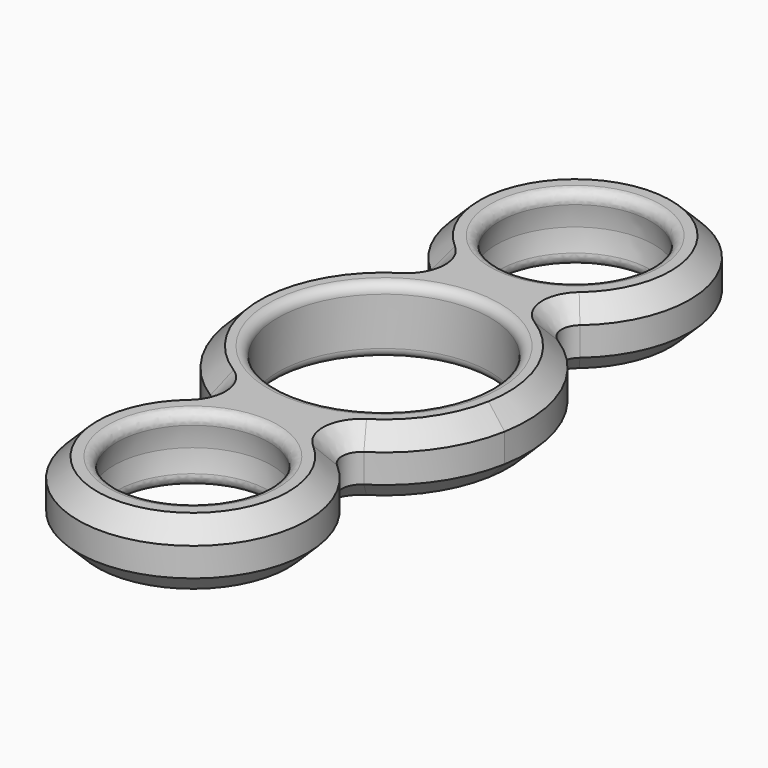
from build123d import *

# Parameters (mm, degrees)
F0_R     = 8.25
F0_R_2   = 11.1
F1_DEPTH = 7
F2_R     = 2
F3_SIZE  = 2
F9_R     = 1


# Not quite as in the source:
# - a pattern or mirror of a feature is missing from the dataset's text; its kind, count and spacing are read off the source's solid
# - a feature names something its author has since deleted; it is built from what else it names


with BuildPart() as f1:
    # F0 (on Top) → F1 (new body)
    with BuildSketch(Plane.XY):
        with BuildLine():
            ThreePointArc((14.7593654246, -2.6760291972), (12.9903810568, 7.5), (5.0621734463, 14.12))
            ThreePointArc((5.0621734463, 14.12), (0, 37), (-5.0621734463, 14.12))
            ThreePointArc((-5.0621734463, 14.12), (-15, 0), (-5.0621734463, -14.12))
            ThreePointArc((-5.0621734463, -14.12), (0, -37), (5.0621734463, -14.12))
            ThreePointArc((5.0621734463, -14.12), (11.4439708028, -9.6971919783), (14.7593654246, -2.6760291972))
        make_face()
        with Locations((0, -25)):
            Circle(F0_R, mode=Mode.SUBTRACT)
        Circle(F0_R_2, mode=Mode.SUBTRACT)
        with Locations((0, 25)):
            Circle(F0_R, mode=Mode.SUBTRACT)
    extrude(amount=F1_DEPTH)

    # F2
    f2_edges = [f1.edges().sort_by_distance(p)[0] for p in [
        (5.062173, -14.12, 3.5),
        (5.062173, 14.12, 3.5),
        (-5.062173, 14.12, 3.5),
        (-5.062173, -14.12, 3.5),
    ]]
    fillet(f2_edges, radius=F2_R)

    # F3
    f3_edges = [f1.edges().sort_by_distance(p)[0] for p in [
        (0, -37, 7),
        (0, -37, 0),
        (15, 0, 7),
        (15, 0, 0),
        (7.104012, 14.217419, 7),
        (7.104012, -14.217419, 7),
        (0, 37, 7),
        (-7.104012, 14.217419, 7),
        (-7.104012, -14.217419, 7),
        (-15, 0, 7),
        (7.104012, 14.217419, 0),
        (7.104012, -14.217419, 0),
        (0, 37, 0),
        (-7.104012, -14.217419, 0),
        (-7.104012, 14.217419, 0),
        (-15, 0, 0),
    ]]
    chamfer(f3_edges, length=F3_SIZE)

    # F7 (on 3pt) → F8 (revolve)
    with BuildSketch(Plane.YZ):
        with BuildLine():
            Line((-32.4707763987, 7), (-33.25, 7))
            Line((-33.25, 7), (-33.25, 3.5))
            ThreePointArc((-33.25, 3.5), (-33.0528381733, 5.2928461605), (-32.4707763987, 7))
        make_face()
        with BuildLine():
            ThreePointArc((-32.4707763987, 0), (-33.0528381733, 1.7071538395), (-33.25, 3.5))
            Line((-33.25, 3.5), (-33.25, 0))
            Line((-33.25, 0), (-32.4707763987, 0))
        make_face()
    f8 = revolve(axis=Axis((0, -25, 3.5), (0, 0, 1)))

    # F8_copies: F8 across plane
    add(f8.mirror(Plane.ZX))

    # F9
    f9_edges = [f1.edges().sort_by_distance(p)[0] for p in [
        (0, -17.529224, 7),
        (0, -17.529224, 0),
        (-11.1, 0, 0),
        (-11.1, 0, 7),
        (0, 17.529224, 7),
        (0, 17.529224, 0),
    ]]
    fillet(f9_edges, radius=F9_R)


solid = f1.part
